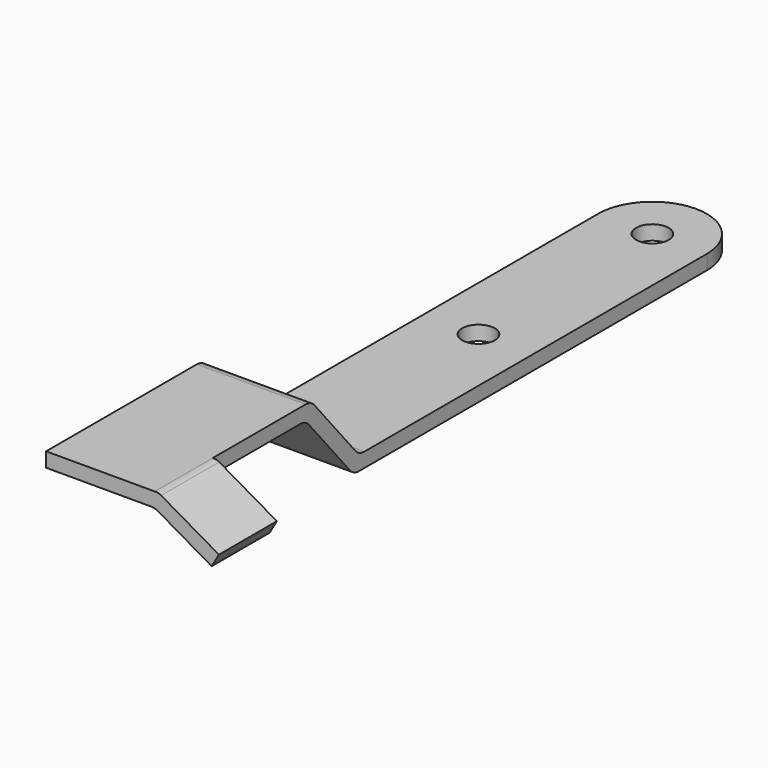
from build123d import *

# Parameters (mm, degrees)
F1_DEPTH     = 2
F3_DEPTH     = 15
F4_W         = 15
F4_H         = 36.1711822092
F5_DEPTH     = 2
F6_W         = 16
F6_H         = 2
F7_DEPTH     = 15
F8_R         = 2
F11_DEPTH    = 10
F12_R        = 2.25
F13_DEPTH    = 25
F14_T1_DEPTH = 10


# Not quite as in the source:
# - a fillet or chamfer that OpenCascade refuses, or shapes differently, is made with other operations: its cross-section is extruded or revolved along the edge and cut away or added


with BuildPart() as f1:
    # F0 (on Top) → F1 (new body)
    with BuildSketch(Plane.XY):
        with BuildLine():
            Line((-7.5, 60), (-7.5, 0))
            Line((-7.5, 0), (7.5, 0))
            Line((7.5, 0), (7.5, 60))
            ThreePointArc((7.5, 60), (0, 67.5), (-7.5, 60))
        make_face()
    extrude(amount=F1_DEPTH)

    # F2 (on face) → F3 (join, through all)
    with BuildSketch(Plane.YZ.offset(7.5)):
        with BuildLine():
            Line((-9.1977466834, 9.85), (-1.5320888862, 0.7144247806))
            ThreePointArc((-1.5320888862, 0.7144247806), (-0.8452365235, 0.1873844259), (0, 0))
            Line((0, 0), (0, 2))
            Line((0, 2), (-7.6656577972, 11.1355752194))
            ThreePointArc((-7.6656577972, 11.1355752194), (-8.3525101599, 11.6626155741), (-9.1977466834, 11.85))
            Line((-9.1977466834, 11.85), (-9.1977466834, 9.85))
        make_face()
    extrude(amount=-F3_DEPTH)

    # F6 (on face) → F7 (join, through all)
    with BuildSketch(Plane(origin=(-7.5, 0, 0), x_dir=(0, -1, 0), z_dir=(-1, 0, 0))):
        with Locations((17.1977466834, 10.85)):
            Rectangle(F6_W, F6_H)
    extrude(amount=-F7_DEPTH)

    # F8
    f8_edges = [f1.edges().sort_by_distance(p)[0] for p in [
        (0, 0, 0),
        (0, 0, 2),
        (0, -9.197747, 11.85),
        (0, -9.197747, 9.85),
    ]]
    fillet(f8_edges, radius=F8_R)

    # F10 (on face) → F11 (join)
    with BuildSketch(Plane.XZ.offset(25.1977466834)):
        with BuildLine():
            Line((-7.5, 9.85), (7.5, 9.85))
            Line((7.5, 9.85), (15.3476885433, 5.319134907))
            Line((15.3476885433, 5.319134907), (16.3476885433, 7.0511857146))
            Line((16.3476885433, 7.0511857146), (8.384588029, 11.6486839401))
            ThreePointArc((8.384588029, 11.6486839401), (7.9574981533, 11.8161493535), (7.5, 11.85))
            Line((7.5, 11.85), (-7.5, 11.85))
            Line((-7.5, 11.85), (-7.5, 9.85))
        make_face()
    extrude(amount=F11_DEPTH)

    # F12 (on face) → F13 (cut)
    with BuildSketch(Plane.XY.offset(2)):
        with Locations((0, 60)):
            Circle(F12_R)
        with Locations((0, 30)):
            Circle(F12_R)
    extrude(amount=-F13_DEPTH, mode=Mode.SUBTRACT)

    # F14: fillet of radius 2 on 1 edges, made by hand

    # F14_s2 → F14_t1 (join)
    with BuildSketch(Plane.XZ.offset(25.1977466834)):
        with BuildLine():
            ThreePointArc((6.9641016151, 9.85), (7.4817397053, 9.7818516526), (7.9641016151, 9.5820508076))
            Line((7.9641016151, 9.5820508076), (7.5, 9.85))
            Line((7.5, 9.85), (6.9641016151, 9.85))
        make_face()
    extrude(amount=F14_T1_DEPTH)


with BuildPart() as f5:
    # F4 (on face) → F5 (new body)
    with BuildSketch(Plane.XY.offset(2)):
        with Locations((0, -25.7512489018)):
            Rectangle(F4_W, F4_H)
    extrude(amount=F5_DEPTH)


solid = f1.part
